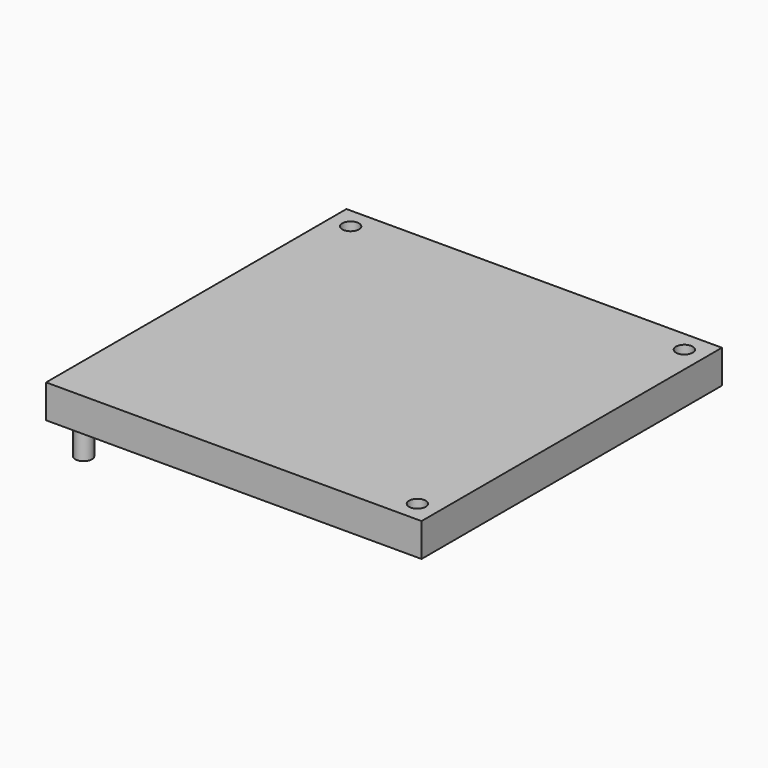
from build123d import *

# Parameters (mm, degrees)
F0_W     = 450
F0_H     = 450
F0_R     = 10
F1_DEPTH = 40
F2_R     = 10
F3_DEPTH = 80


# Not quite as in the source:
# - the program builds the solid bodies; features that only make, move or delete a surface that nothing else refers to are left out


with BuildPart() as f1:
    # F0 (on Top) → F1 (new body)
    with BuildSketch(Plane.XY):
        Rectangle(F0_W, F0_H)
        with Locations((-200, -200)):
            Circle(F0_R, mode=Mode.SUBTRACT)
        with Locations((200, -200)):
            Circle(F0_R, mode=Mode.SUBTRACT)
        with Locations((-200, 200)):
            Circle(F0_R, mode=Mode.SUBTRACT)
        with Locations((200, 200)):
            Circle(F0_R, mode=Mode.SUBTRACT)
    extrude(amount=F1_DEPTH)

    # F2 (on face) → F3 (join)
    with BuildSketch(Plane.XY.offset(40)):
        with Locations((-200, -200)):
            Circle(F2_R)
    extrude(amount=-F3_DEPTH)


solid = f1.part
